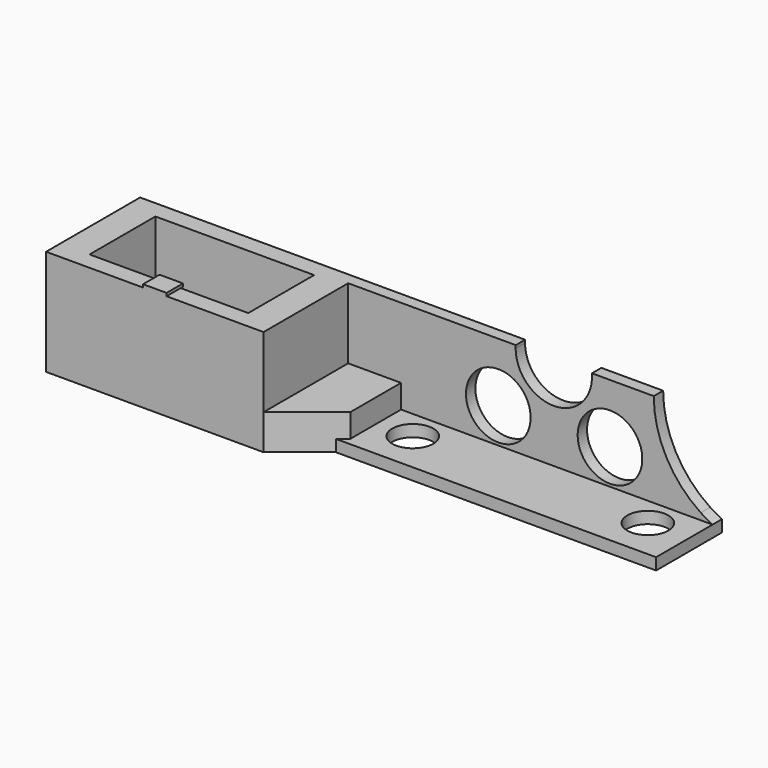
from build123d import *

# Parameters (mm, degrees)
F0_W     = 18.5
F0_H     = 10
F0_W_2   = 13.5
F0_H_2   = 7
F1_DEPTH = 9
F3_DEPTH = 3
F2_W     = 25
F2_H     = 1
F2_H_2   = 5
F2_R     = 1.75
F4_DEPTH = 1
F5_R     = 2.75
F6_DEPTH = 1
F7_W     = 2
F7_H     = 1.75
F8_DEPTH = 0.25


with BuildPart() as f1:
    # F0 (on Top) → F1 (new body)
    with BuildSketch(Plane.XY):
        Rectangle(F0_W, F0_H)
        Rectangle(F0_W_2, F0_H_2, mode=Mode.SUBTRACT)
    extrude(amount=F1_DEPTH)

    # F2 (on face) → F3 (join)
    with BuildSketch(Plane(origin=(0, 0, 0), x_dir=(1, 0, 0), z_dir=(0, 0, -1))):
        Polygon((9.25, -5), (13.75, -5), (13.75, 1.4), (13, 2), (9.25, 5), align=None)
    extrude(amount=-F3_DEPTH)

    # F2 (on face) → F4 (join)
    with BuildSketch(Plane(origin=(0, 0, 0), x_dir=(1, 0, 0), z_dir=(0, 0, -1))):
        Polygon((13.75, -5), (14.25, -5), (14.25, -4), (14.25, 1), (13.75, 1.4), align=None)
        Polygon((39.25, -4), (39.25, -5), (40.25, -5), (40.25, 2), (13, 2), (13.75, 1.4), (14.25, 1), (39.25, 1), align=None)
        with Locations((26.75, -4.5)):
            Rectangle(F2_W, F2_H)
        with Locations((26.75, -1.5)):
            Rectangle(F2_W, F2_H_2)
        with Locations((16.75, -1.5)):
            Circle(F2_R, mode=Mode.SUBTRACT)
        with Locations((36.75, -1.5)):
            Circle(F2_R, mode=Mode.SUBTRACT)
    extrude(amount=-F4_DEPTH)

    # F5 (on face) → F6 (join)
    with BuildSketch(Plane(origin=(0, 5, 0), x_dir=(-1, 0, 0), z_dir=(0, 1, 0))):
        Polygon((-13.75, 1), (-14.25, 1), (-39.25, 1), (-40.25, 1), (-40.25, 0), (9.25, 0), (9.25, 9), (-9.25, 9), (-9.25, 3), (-9.25, 1), align=None)
        with BuildLine():
            Line((-39.25, 1), (-14.25, 1))
            Line((-14.25, 1), (-14.25, 9))
            Line((-14.25, 9), (-23.5096296508, 9))
            ThreePointArc((-23.5096296508, 9), (-23.502408305, 8.8750926958), (-23.5, 8.75))
            ThreePointArc((-23.5, 8.75), (-26.8750926958, 5.502408305), (-29.9903703492, 9))
            Line((-29.9903703492, 9), (-35.25, 9))
            ThreePointArc((-35.25, 9), (-36.3135467206, 4.7809953781), (-39.25, 1.5703297516))
            Line((-39.25, 1.5703297516), (-39.25, 1))
        make_face()
        with Locations((-31.525, 3.975)):
            Circle(F5_R, mode=Mode.SUBTRACT)
        with Locations((-22.025, 3.975)):
            Circle(F5_R, mode=Mode.SUBTRACT)
        Polygon((-14.25, 9), (-14.25, 1), (-13.75, 1), (-13.75, 3), (-9.25, 3), (-9.25, 9), align=None)
        with BuildLine():
            Line((-40.25, 1), (-39.25, 1))
            Line((-39.25, 1), (-39.25, 1.5703297516))
            ThreePointArc((-39.25, 1.5703297516), (-39.7407688872, 1.2689793045), (-40.25, 1))
        make_face()
    extrude(amount=-F6_DEPTH)

    # F7 (on face) → F8 (join)
    with BuildSketch(Plane.XY.offset(9)):
        with Locations((0, -4.125)):
            Rectangle(F7_W, F7_H)
    extrude(amount=F8_DEPTH)


solid = f1.part
